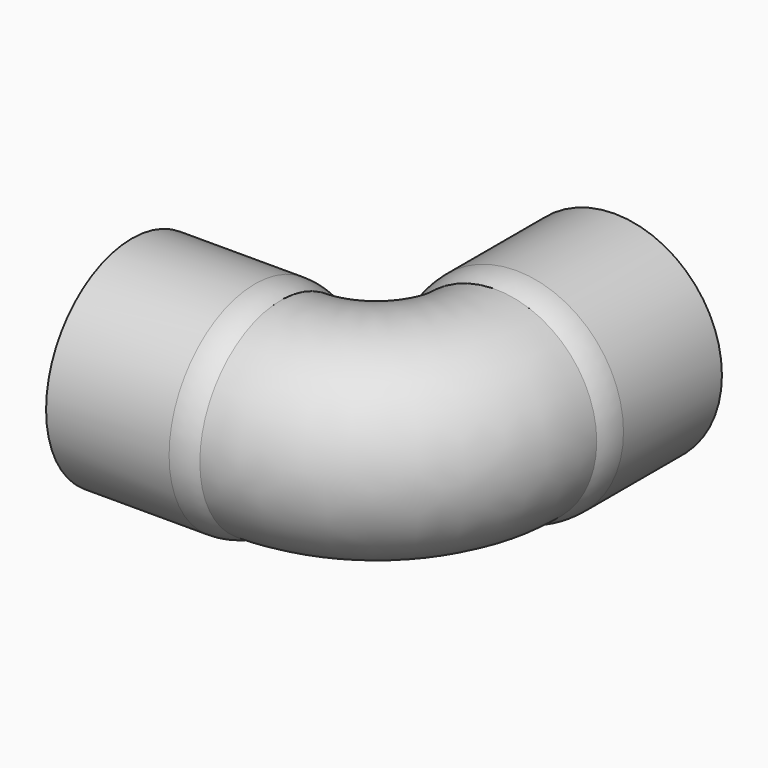
from build123d import *

# Parameters (mm, degrees)
F0_R     = 8.5
F0_R_2   = 7.5
F1_ANGLE = 90
F2_R     = 9
F2_R_2   = 7.25
F3_DEPTH = 12.5
F4_R     = 9
F4_R_2   = 7.25
F5_DEPTH = 12.5


# Not quite as in the source:
# - a fillet or chamfer that OpenCascade refuses, or shapes differently, is made with other operations: its cross-section is extruded or revolved along the edge and cut away or added


with BuildPart() as f1:
    # F0 (on Front) → F1 (revolve)
    with BuildSketch(Plane.XZ):
        Circle(F0_R)
        Circle(F0_R_2, mode=Mode.SUBTRACT)
    revolve(axis=Axis((-10, 0, 0.1811354887), (0, 0, -1)), revolution_arc=F1_ANGLE)

    # F2 (on Front) → F3 (join)
    with BuildSketch(Plane.XZ):
        Circle(F2_R)
        Circle(F2_R_2, mode=Mode.SUBTRACT)
    extrude(amount=-F3_DEPTH)

    # F4 (on face) → F5 (join)
    with BuildSketch(Plane(origin=(-10, 0, 0), x_dir=(0, -1, 0), z_dir=(-1, 0, 0))):
        with Locations((10, 0)):
            Circle(F4_R)
        with Locations((10, 0)):
            Circle(F4_R_2, mode=Mode.SUBTRACT)
    extrude(amount=F5_DEPTH)

    # F6: fillet of radius 5 on 2 edges, made by hand

    # F6_s1 → F6_t2 (revolve, cut)
    with BuildSketch(Plane.XY):
        with BuildLine():
            ThreePointArc((-12.1794494718, -19), (-11.061415483, -18.8733971724), (-10, -18.5))
            Line((-10, -18.5), (-10, -19))
            Line((-10, -19), (-12.1794494718, -19))
        make_face()
    revolve(axis=Axis((-10, -10, 0), (-1, 0, 0)), mode=Mode.SUBTRACT)

    # F6_s3 → F6_t4 (revolve, cut)
    with BuildSketch(Plane.XY):
        with BuildLine():
            ThreePointArc((8.5, 0), (8.8733971724, 1.061415483), (9, 2.1794494718))
            Line((9, 2.1794494718), (9, 0))
            Line((9, 0), (8.5, 0))
        make_face()
    revolve(axis=Axis((0, 0, 0), (0, -1, 0)), mode=Mode.SUBTRACT)


solid = f1.part
